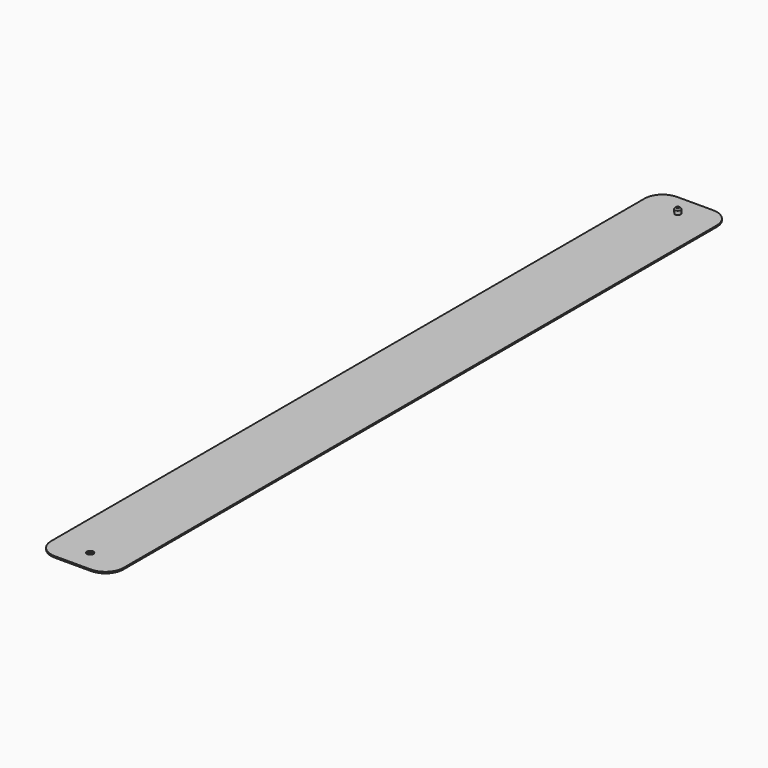
from build123d import *

# Parameters (mm, degrees)
F1_DEPTH = 0.4
F2_R     = 0.75
F3_DEPTH = 1.5
F3_TAPER = -3
F5_D     = 1.8


# Not quite as in the source:
# - a fillet or chamfer that OpenCascade refuses, or shapes differently, is made with other operations: its cross-section is extruded or revolved along the edge and cut away or added


with BuildPart() as f1:
    # F0 (on Top) → F1 (new body)
    with BuildSketch(Plane.XY):
        with BuildLine():
            Line((-6.5418671444, 67.6613259315), (-16.5418671444, 67.6613259315))
            ThreePointArc((-16.5418671444, 67.6613259315), (-20.0774010503, 66.1968598375), (-21.5418671444, 62.6613259315))
            Line((-21.5418671444, 62.6613259315), (-21.5418671444, -142.3386740685))
            ThreePointArc((-21.5418671444, -142.3386740685), (-20.0774010503, -145.8742079744), (-16.5418671444, -147.3386740685))
            Line((-16.5418671444, -147.3386740685), (-6.5418671444, -147.3386740685))
            ThreePointArc((-6.5418671444, -147.3386740685), (-3.0063332385, -145.8742079744), (-1.5418671444, -142.3386740685))
            Line((-1.5418671444, -142.3386740685), (-1.5418671444, 62.6613259315))
            ThreePointArc((-1.5418671444, 62.6613259315), (-3.0063332385, 66.1968598375), (-6.5418671444, 67.6613259315))
        make_face()
    extrude(amount=F1_DEPTH)

    # F2 (on face) → F3 (join)
    with BuildSketch(Plane.XY.offset(0.4)):
        with Locations((-11.5418671444, 61.6613259315)):
            Circle(F2_R)
    extrude(amount=F3_DEPTH, taper=F3_TAPER)

    # F4: chamfer of 0.4 on 1 edges, made by hand

    # F4_s1 → F4_t2 (revolve, cut)
    with BuildSketch(Plane.XZ.offset(-61.6613259315)):
        Polygon((-10.734189858, 1.5005481861), (-11.1132554755, 1.9), (-10.7132554755, 1.9), align=None)
    revolve(axis=Axis((-11.5418671444, 61.6613259315, 1.9), (0, 0, -1)), mode=Mode.SUBTRACT)

    # F5 (through all)
    with Locations(Plane.XY.offset(0.4)):
        with Locations((-11.5418671444, -141.3386740685)):
            Hole(F5_D / 2)


solid = f1.part
